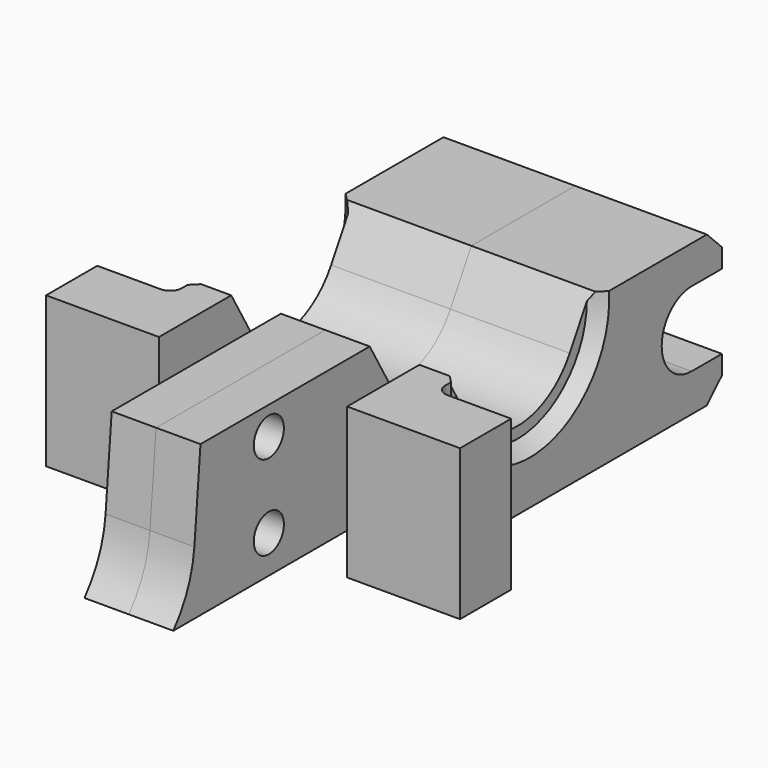
from build123d import *

# Parameters (mm, degrees)
F1_DEPTH  = 50.8
F2_R      = 3.9624
F3_SIZE   = 6.35
F5_DEPTH  = 44.451
F7_D      = 13.0302
F9_DEPTH  = 69.851
F10_R     = 29.21
F11_DEPTH = 29.591
F12_SIZE  = 4.19099
F14_DEPTH = 14.9870001
F16_DEPTH = 16.764
F17_R     = 6.35
F18_DEPTH = 69.851


# Not quite as in the source:
# - a fillet or chamfer is up to 0.001 mm smaller than in the source, because OpenCascade refuses the exact size


with BuildPart() as f1:
    # F0 (on Top) → F1 (new body)
    with BuildSketch(Plane.XY):
        Polygon((44.45, 120.65), (0, 120.65), (0, 0), (0, -21.59), (0, -73.9648), (14.986, -73.9648), (14.986, 26.2809675187), (31.75, 26.2809675187), (31.75, -21.59), (69.85, -21.59), (69.85, 0), (44.45, 0), align=None)
    extrude(amount=F1_DEPTH)

    # F2
    f2_edges = [f1.edges().sort_by_distance(p)[0] for p in [
        (44.45, 0, 25.4),
        (14.986, 26.280968, 25.4),
        (31.75, 26.280968, 25.4),
    ]]
    fillet(f2_edges, radius=F2_R)

    # F3
    f3_edges = [f1.edges().sort_by_distance(p)[0] for p in [
        (22.225, 120.65, 50.8),
        (22.225, 120.65, 0),
    ]]
    chamfer(f3_edges, length=F3_SIZE)

    # F4 (on face) → F5 (cut, through all)
    with BuildSketch(Plane.YZ.offset(44.45)):
        with BuildLine():
            Line((120.65, 38.0365), (107.8865, 38.0365))
            ThreePointArc((107.8865, 38.0365), (95.25, 25.4), (107.8865, 12.7635))
            Line((107.8865, 12.7635), (120.65, 12.7635))
            Line((120.65, 12.7635), (120.65, 38.0365))
        make_face()
    extrude(amount=-F5_DEPTH, mode=Mode.SUBTRACT)

    # F7 (through all)
    with Locations(Plane.YZ.offset(69.85)):
        with Locations((7.62, 12.954)):
            Hole(F7_D / 2)

    # F8 (on face) → F9 (cut, through all)
    with BuildSketch(Plane(origin=(0, 0, 0), x_dir=(0, -1, 0), z_dir=(-1, 0, 0))):
        with BuildLine():
            Line((-8.8916366414, 50.8), (-70.4833633586, 50.8))
            Line((-70.4833633586, 50.8), (-61.6845452561, 35.56))
            ThreePointArc((-61.6845452561, 35.56), (-39.6875, 22.86), (-17.6904547439, 35.56))
            Line((-17.6904547439, 35.56), (-8.8916366414, 50.8))
        make_face()
    extrude(amount=-F9_DEPTH, mode=Mode.SUBTRACT)

    # F10 (on face) → F11 (cut)
    with BuildSketch(Plane.YZ.offset(69.85)):
        with Locations((39.6875, 48.26)):
            Circle(F10_R)
    extrude(amount=-F11_DEPTH, mode=Mode.SUBTRACT)

    # F12 (size 4.191 in the source; OpenCascade refuses exactly that, so slightly less here)
    f12_edges = [f1.edges().sort_by_distance(p)[0] for p in [
        (44.45, 39.6875, 19.05),
    ]]
    chamfer(f12_edges, length=F12_SIZE)

    # F13 (on face) → F14 (cut, through all)
    with BuildSketch(Plane.YZ.offset(14.986)):
        with BuildLine():
            Line((-73.9648, 50.8), (-73.9648, 0))
            ThreePointArc((-73.9648, 0), (-67.8661098873, 9.9669221787), (-65.0748, 21.3133818873))
            Line((-65.0748, 21.3133818873), (-62.4950551894, 50.8))
            Line((-62.4950551894, 50.8), (-73.9648, 50.8))
        make_face()
    extrude(amount=-F14_DEPTH, mode=Mode.SUBTRACT)

    # F15 (on face) → F16 (cut, through all)
    with BuildSketch(Plane.YZ.offset(14.986)):
        Polygon((11.9264439221, 19.6698105436), (22.8565887415, 19.6698105436), (41.9241071546, 38.7373289567), (11.9264439221, 38.7373289567), align=None)
    extrude(amount=F16_DEPTH, mode=Mode.SUBTRACT)

    # F17 (on face) → F18 (cut, through all)
    with BuildSketch(Plane(origin=(0, 0, 0), x_dir=(0, -1, 0), z_dir=(-1, 0, 0))):
        with Locations((33.655, 12.7)):
            Circle(F17_R)
        with Locations((33.655, 41.275)):
            Circle(F17_R)
    extrude(amount=-F18_DEPTH, mode=Mode.SUBTRACT)


with BuildPart() as f19_1:
    # F19: instance of F1
    add(f1.part.mirror(Plane.YZ))


solid = Compound([f1.part, f19_1.part])
